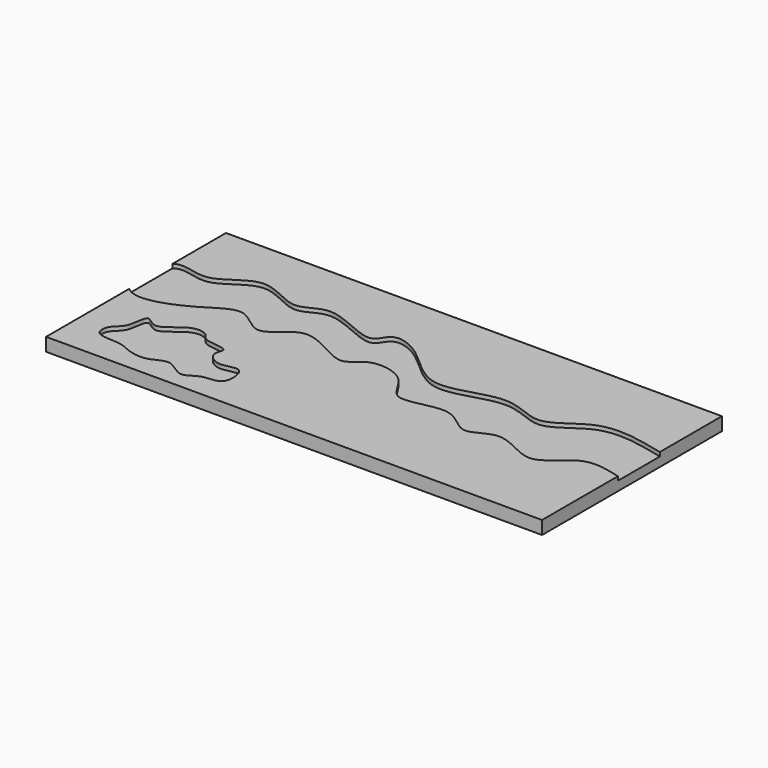
from build123d import *

# Parameters (mm, degrees)
F0_W     = 1500
F0_H     = 680
F1_DEPTH = 40
F2_R     = 3
F3_DEPTH = 12
F5_DEPTH = 12
F7_DEPTH = 12
F8_R     = 3
F9_DEPTH = 12


with BuildPart() as f1:
    # F0 (on Top) → F1 (new body)
    with BuildSketch(Plane.XY):
        with Locations((-750, 340)):
            Rectangle(F0_W, F0_H)
    extrude(amount=F1_DEPTH)

    # F2 (on face) → F3 (cut)
    with BuildSketch(Plane(origin=(0, 0, 0), x_dir=(1, 0, 0), z_dir=(0, 0, -1))):
        with Locations((-1480, -20)):
            Circle(F2_R)
    extrude(amount=-F3_DEPTH, mode=Mode.SUBTRACT)

    # F4 (on face) → F5 (cut)
    with BuildSketch(Plane.XY.offset(40)):
        with BuildLine():
            add(Edge.make_bspline(
                [(0, 286.4934802055), (0, 339.4372363885), (0, 392.3809925715), (0, 445.3247487545)],
                knots=[0, 0, 0, 0, 158.831268549, 158.831268549, 158.831268549, 158.831268549], degree=3))
            add(Edge.make_bspline(
                [(0, 445.3247487545), (-71.3026814156, 462.6306856263), (-201.9329061945, 494.3360630214), (-317.2378699702, 357.8812187635), (-446.7670483399, 461.0443250548), (-644.4835324668, 342.5172822574), (-758.9975475315, 492.9974148266), (-869.9027366953, 530.3244908478), (-887.2539027471, 436.8064706214), (-1062.3063047285, 558.5374533926), (-1138.4438056143, 459.5841560087), (-1277.8049893694, 578.348863664), (-1385.0565915133, 438.9739778644), (-1475.0237093397, 498.061505044), (-1500, 477.6328206062)],
                knots=[0, 0, 0, 0, 0.0471608855, 0.0864011977, 0.1243763857, 0.1704285887, 0.2138514082, 0.2455973931, 0.2693538935, 0.3120725393, 0.3441713118, 0.3829340036, 0.4219710198, 0.4561412375, 0.4561412375, 0.4561412375, 0.4561412375], degree=3))
            add(Edge.make_bspline(
                [(-1500, 315.3073489666), (-1500, 369.4158395131), (-1500, 423.5243300597), (-1500, 477.6328206062)],
                knots=[0, 0, 0, 0, 162.3254716396, 162.3254716396, 162.3254716396, 162.3254716396], degree=3))
            add(Edge.make_bspline(
                [(-1500, 315.3073489666), (-1462.2600291653, 276.3418664841), (-1312.4238194047, 332.288384945), (-1215.7717532273, 419.458281524), (-1122.6460566347, 297.0338326998), (-1038.5933218584, 447.4185705032), (-877.0930588694, 303.0847497239), (-834.1231388754, 393.2153868752), (-699.644533812, 371.2777207184), (-675.1018374932, 242.3278334168), (-509.3298165671, 327.6927496618), (-434.4092269545, 211.2526621407), (-344.7647124023, 306.3571113689), (-211.8966957667, 185.2725036422), (-125.0126714016, 320.6591881695), (-41.6853977312, 297.8860143325), (0, 286.4934802055)],
                knots=[0.4986966286, 0.4986966286, 0.4986966286, 0.4986966286, 0.5435361072, 0.5799004761, 0.6127047397, 0.6476288977, 0.6895773278, 0.7169601646, 0.7518811924, 0.784411176, 0.8238440199, 0.8571376432, 0.8886822223, 0.9272958417, 0.9636289342, 1, 1, 1, 1], degree=3))
        make_face()
    extrude(amount=-F5_DEPTH, mode=Mode.SUBTRACT)

    # F6 (on face) → F7 (cut)
    with BuildSketch(Plane.XY.offset(40)):
        with BuildLine():
            add(Edge.make_bspline(
                [(-1334.7696065903, 206.4833641052), (-1313.2105290239, 204.2148342911), (-1271.0010693131, 260.2903304188), (-1209.7086044003, 251.2161388238), (-1202.0827161363, 216.5365177186), (-1114.4083487148, 221.9710931235), (-1147.9717713113, 178.169190651), (-1095.2906259726, 132.768035853), (-1026.1400400498, 175.9872446047), (-1016.1644902216, 64.4883972315), (-1090.696332941, 81.1539802015), (-1131.5755110793, 30.7430863353), (-1189.8546428408, 96.851268769), (-1240.1483248307, 52.7781486986), (-1305.1202383489, 63.9218007253), (-1340.592884341, 88.2474203251), (-1424.607066336, 79.3111891901), (-1420.549922877, 139.0681343602), (-1378.2165282406, 156.8384289437), (-1381.3821812047, 248.9236486972), (-1350.0595465471, 208.092230929), (-1334.7696065903, 206.4833641052)],
                knots=[0, 0, 0, 0, 0.0654118182, 0.1167160778, 0.1561764291, 0.2136874293, 0.2533446011, 0.306046933, 0.3611581397, 0.4200638456, 0.4749436617, 0.5264375146, 0.584433548, 0.6384389443, 0.6947224268, 0.7440524576, 0.8042869701, 0.8490166151, 0.8979247009, 0.9536092039, 1, 1, 1, 1], degree=3))
        make_face()
    extrude(amount=-F7_DEPTH, mode=Mode.SUBTRACT)

    # F8 (on face) → F9 (cut)
    with BuildSketch(Plane(origin=(0, 0, 0), x_dir=(1, 0, 0), z_dir=(0, 0, -1))):
        with Locations((-1480, -660)):
            Circle(F8_R)
        with Locations((-20, -660)):
            Circle(F8_R)
        with Locations((-20, -20)):
            Circle(F8_R)
    extrude(amount=-F9_DEPTH, mode=Mode.SUBTRACT)


solid = f1.part
